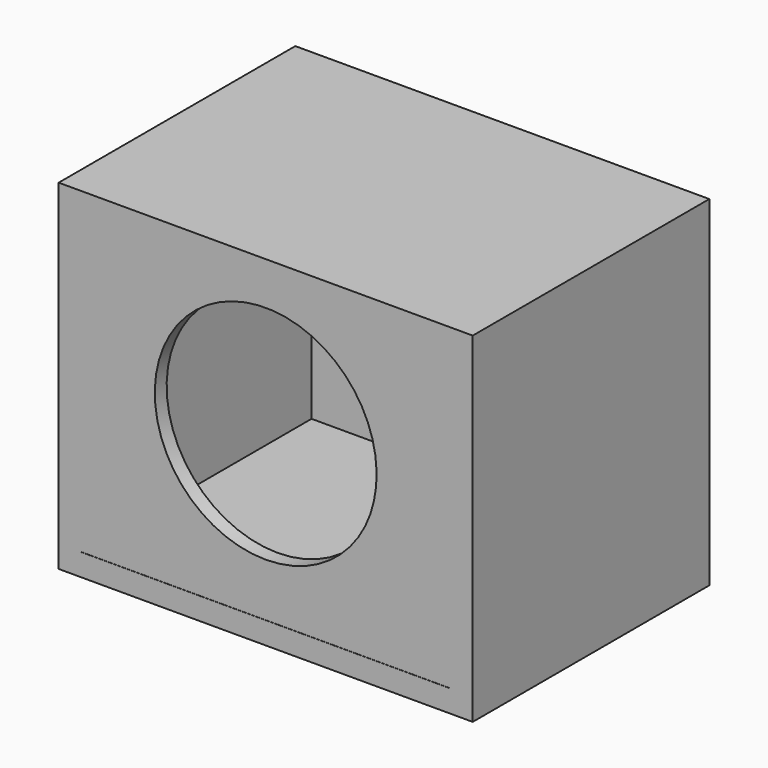
from build123d import *

# Parameters (mm, degrees)
F1_DEPTH = 20
F5_DEPTH = 1
F7_DEPTH = 2


# Not quite as in the source:
# - a feature names something its author has since deleted; it is built from what else it names


with BuildPart() as f1:
    # F0 (on Front) → F1 (new body, symmetric)
    with BuildSketch(Plane.XZ):
        Polygon((-25, -3.4681803342), (-25, 36.5318196658), (25, 36.5318196658), (25, 26.5318196658), (28, 26.5318196658), (28, 39.5318196658), (-28, 39.5318196658), (-28, -6.4681803342), (0, -6.4681803342), (0, -3.4681803342), align=None)
        Polygon((28, 26.5318196658), (25, 26.5318196658), (25, -3.4681803342), (0, -3.4681803342), (0, -6.4681803342), (28, -6.4681803342), align=None)
    extrude(amount=F1_DEPTH, both=True)

    # F4 (on offset) → F5 (join)
    with BuildSketch(Plane.XZ.offset(-20)):
        Polygon((25, -3.5996623058), (25, 36.4003376942), (-25, 36.4003376942), (-25, -3.5996623058), (0, -3.5996623058), align=None)
        with BuildLine():
            ThreePointArc((5, 19.2190613598), (3.5355339059, 15.6835274538), (0, 14.2190613598))
            ThreePointArc((0, 14.2190613598), (-5, 19.2190613598), (0, 24.2190613598))
            ThreePointArc((0, 24.2190613598), (3.5355339059, 22.7545952657), (5, 19.2190613598))
        make_face(mode=Mode.SUBTRACT)
    extrude(amount=F5_DEPTH)

    # F6 (on offset) → F7 (join)
    with BuildSketch(Plane.XZ.offset(20)):
        Polygon((-25, 36.5481637139), (-25, -3.4518362861), (0, -3.4518362861), (25, -3.4518362861), (25, 36.5481637139), align=None)
        with BuildLine():
            ThreePointArc((15, 18.7427662313), (10.6066017178, 8.1361645135), (0, 3.7427662313))
            ThreePointArc((0, 3.7427662313), (-10.6066017178, 29.3493679491), (15, 18.7427662313))
        make_face(mode=Mode.SUBTRACT)
    extrude(amount=-F7_DEPTH)


solid = f1.part
